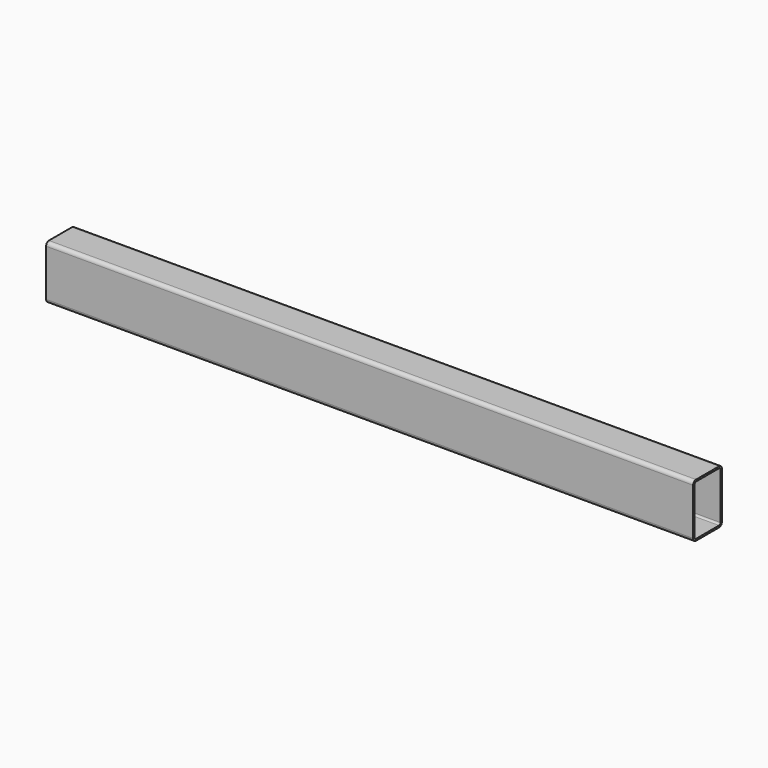
from build123d import *

# Parameters (mm, degrees)
F1_DEPTH = 1800


# Not quite as in the source:
# - ends of sketch curves that miss each other by under 0.0002 mm in the source are joined


with BuildPart() as f1:
    # F0 (on Right) → F1 (new body)
    with BuildSketch(Plane.YZ):
        with BuildLine():
            ThreePointArc((50, 65), (47.0710678119, 72.0710678119), (40, 75))
            Line((40, 75), (-40, 75))
            ThreePointArc((-40, 75), (-47.0710678119, 72.0710678119), (-50, 65))
            Line((-50, 65), (-50, -65))
            ThreePointArc((-50, -65), (-47.0710678119, -72.0710678119), (-40, -75))
            Line((-40, -75), (40, -75))
            ThreePointArc((40, -75), (47.0710678119, -72.0710678119), (50, -65))
            Line((50, -65), (50, 65))
        make_face()
        with BuildLine():
            ThreePointArc((40, 70.0000021271), (43.53553541, 68.53553541), (45.0000021271, 65))
            Line((45.0000021271, 65), (45, -65))
            ThreePointArc((45, -65), (43.53553541, -68.53553541), (40, -70.0000021271))
            Line((40, -70.0000021271), (-40, -70))
            ThreePointArc((-40, -70), (-43.53553541, -68.53553541), (-45.0000021271, -65))
            Line((-45.0000021271, -65), (-45, 65))
            ThreePointArc((-45, 65), (-43.53553541, 68.53553541), (-40, 70.0000021271))
            Line((-40, 70.0000021271), (40, 70.0000021271))
        make_face(mode=Mode.SUBTRACT)
    extrude(amount=F1_DEPTH)


solid = f1.part
